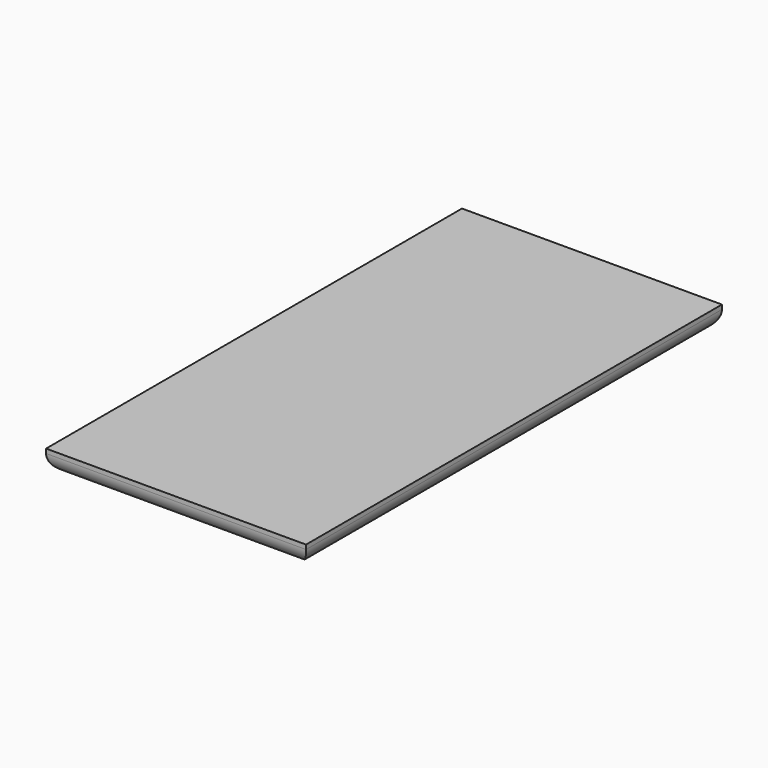
from build123d import *

# Parameters (mm, degrees)
F1_DEPTH = 76.2
F2_DEPTH = 6.35
F3_R     = 5.08


# Not quite as in the source:
# - the program builds the solid bodies; features that only make, move or delete a surface that nothing else refers to are left out


with BuildPart() as f1:
    # F0 (on Front) → F1 (new body, symmetric)
    with BuildSketch(Plane.XZ):
        Polygon((34.29, -3.175), (38.1, -3.175), (38.1, 3.175), (-38.1, 3.175), (-38.1, -3.175), (-34.29, -3.175), align=None)
    extrude(amount=F1_DEPTH, both=True)

    # F0 (on Front) → F2 (join)
    with BuildSketch(Plane.XZ):
        Polygon((34.29, -3.175), (38.1, -3.175), (38.1, 3.175), (-38.1, 3.175), (-38.1, -3.175), (-34.29, -3.175), align=None)
    extrude(amount=F2_DEPTH)

    # F3
    f3_edges = [f1.edges().sort_by_distance(p)[0] for p in [
        (38.1, 0, -3.175),
        (0, -76.2, -3.175),
        (-38.1, 0, -3.175),
        (0, 76.2, -3.175),
    ]]
    fillet(f3_edges, radius=F3_R)


solid = f1.part
